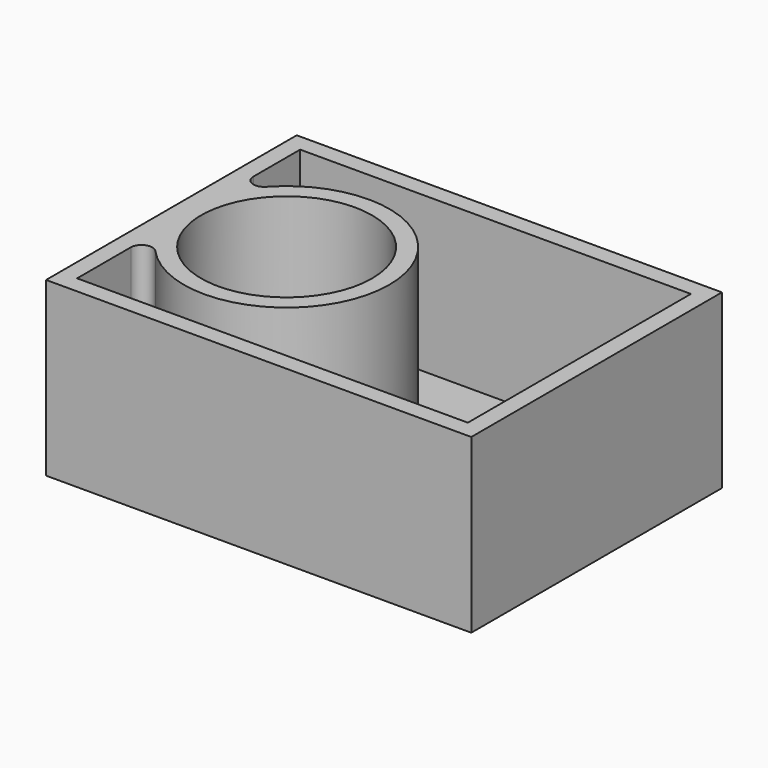
from build123d import *

# Parameters (mm, degrees)
F0_W     = 62.6746565104
F0_H     = 46.1766123772
F0_R     = 12.6048441678
F1_DEPTH = 25.4
F2_T     = -2.54
F3_R     = 1.5875


with BuildPart() as f1:
    # F0 (on Top) → F1 (new body)
    with BuildSketch(Plane.XY):
        with Locations((31.3373282552, 23.0883061886)):
            Rectangle(F0_W, F0_H)
        with Locations((16.4661593735, 23.7301085144)):
            Circle(F0_R, mode=Mode.SUBTRACT)
    extrude(amount=F1_DEPTH)

    # F2
    f2_openings = [f1.faces().sort_by_distance(p)[0] for p in [
        (34.436685, 22.954546, 25.4),
    ]]
    offset(amount=F2_T, openings=f2_openings)

    # F3
    f3_edges = [f1.edges().sort_by_distance(p)[0] for p in [
        (2.54, 29.682284, 13.97),
        (2.54, 17.777933, 13.97),
    ]]
    fillet(f3_edges, radius=F3_R)


solid = f1.part
